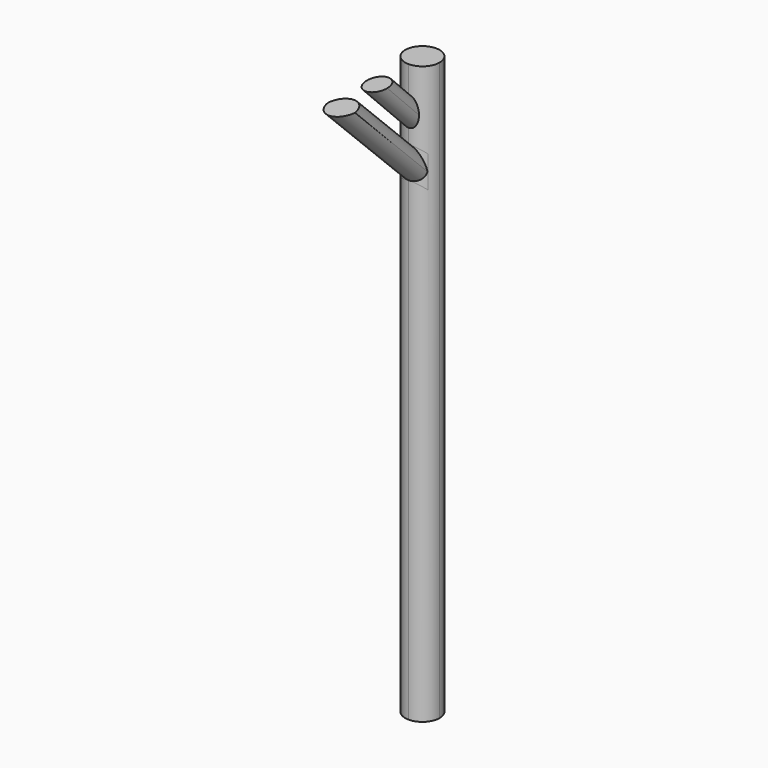
from build123d import *

# Parameters (mm, degrees)
F1_DEPTH     = 63.5
F2_DEPTH     = 38.1
F3_DEPTH     = 50.8
F4_T1_DEPTH  = 2451.0995000004
F4_T6_DEPTH  = 2451.0995000004
F4_T12_DEPTH = 2451.0995000004
F4_T18_DEPTH = 2451.0995000004
F4_T25_DEPTH = 2451.0995000004
F4_T31_DEPTH = 2451.0995000004
F4_T37_DEPTH = 2451.0995000004
F4_T43_DEPTH = 2451.0995000004
F4_T49_DEPTH = 2451.0995000004
F4_T56_DEPTH = 2451.0995000004
F4_T62_DEPTH = 2451.0995000004
F5_R         = 38.09999
F6_T3_DEPTH  = 804.0537236545
F6_S4_R      = 63.5000000002
F6_T5_DEPTH  = 430
F6_T8_DEPTH  = 804.0537236545
F6_S9_R      = 63.5000000002
F6_T10_DEPTH = 430
F6_T13_DEPTH = 641.6247372202
F6_S14_R     = 63.5000000002
F6_T15_DEPTH = 349
F6_T18_DEPTH = 641.6247372202
F6_S19_R     = 63.5000000002
F6_T20_DEPTH = 349
F6_T23_DEPTH = 641.6247372202
F6_S24_R     = 63.5000000002
F6_T25_DEPTH = 349
F6_T28_DEPTH = 641.6247372202
F6_S29_R     = 63.5000000002
F6_T30_DEPTH = 349
F6_T33_DEPTH = 804.0537236545
F6_S34_R     = 63.5000000002
F6_T35_DEPTH = 430
F6_T38_DEPTH = 804.0537236545
F6_S39_R     = 63.5000000002
F6_T40_DEPTH = 430


# Not quite as in the source:
# - a fillet or chamfer that OpenCascade refuses, or shapes differently, is made with other operations: its cross-section is extruded or revolved along the edge and cut away or added
# - a fillet or chamfer is up to 0.001 mm smaller than in the source, because OpenCascade refuses the exact size


with BuildPart() as f1:
    # F0 (on Right) → F1 (new body, symmetric)
    with BuildSketch(Plane.YZ):
        Polygon((-127, 1755.4620370299), (-127, 0), (0, 0), (0, 2133.6), (-127, 2133.6), (-127, 2034.3245418301), (-127, 1926.4060574944), (-127, 1872.7545669842), align=None)
    extrude(amount=F1_DEPTH, both=True)

    # F0 (on Right) → F3 (join, symmetric)
    with BuildSketch(Plane.YZ):
        Polygon((-495.5889745507, 2116.2556735062), (-127, 1755.4620370299), (-127, 1872.7545669842), (-379.5134473118, 2119.9275732464), align=None)
    extrude(amount=F3_DEPTH, both=True)

    # F4: fillet of radius 63.5 on 4 edges, made by hand

    # F4_s2 → F4_t1 (cut)
    with BuildSketch(Plane.XY.offset(-158.7497500002)):
        with BuildLine():
            ThreePointArc((-63.5001, -63.4999), (-44.9013806053, -18.5986193947), (-0.0001, 0.0001))
            Line((-0.0001, 0.0001), (-0.0001, 1.2701))
            Line((-0.0001, 1.2701), (-64.77, 1.27))
            Line((-64.77, 1.27), (-64.7701, -63.4999))
            Line((-64.7701, -63.4999), (-63.5001, -63.4999))
        make_face()
        with BuildLine():
            ThreePointArc((63.5001, -63.4999), (44.9013806053, -18.5986193947), (0.0001, 0.0001))
            Line((0.0001, 0.0001), (0.0001, 1.2701))
            Line((0.0001, 1.2701), (64.77, 1.27))
            Line((64.77, 1.27), (64.7701, -63.4999))
            Line((64.7701, -63.4999), (63.5001, -63.4999))
        make_face()
    extrude(amount=F4_T1_DEPTH, mode=Mode.SUBTRACT)


with BuildPart() as f2:
    # F0 (on Right) → F2 (new body, symmetric)
    with BuildSketch(Plane.YZ):
        Polygon((-326.3924083134, 2126.3731611819), (-127, 1926.4060574944), (-127, 2034.3245418301), (-220.5952878332, 2128.1895930882), align=None)
    extrude(amount=F2_DEPTH, both=True)

    # F5 (radius 38.1 in the source; OpenCascade refuses exactly that, so slightly less here)
    f5_edges = [f2.edges().sort_by_distance(p)[0] for p in [
        (-38.1, -226.696204, 2026.389609),
        (-38.1, -173.797644, 2081.257067),
        (38.1, -173.797644, 2081.257067),
        (38.1, -226.696204, 2026.389609),
    ]]
    fillet(f5_edges, radius=F5_R)


with BuildPart() as f4_tool4:
    # F4_s5 → F4_t6 (new body)
    with BuildSketch(Plane.XY.offset(2292.3497500002)):
        with BuildLine():
            ThreePointArc((-0.0001, -127.0001), (-44.9013806053, -108.4013806053), (-63.5001, -63.5001))
            Line((-63.5001, -63.5001), (-64.7701, -63.5001))
            Line((-64.7701, -63.5001), (-64.77, -128.27))
            Line((-64.77, -128.27), (-0.0001, -128.2701))
            Line((-0.0001, -128.2701), (-0.0001, -127.0001))
        make_face()
    extrude(amount=-F4_T6_DEPTH)

    split(bisect_by=Plane(origin=(0, 874.0205617241, 892.9047245081), x_dir=(1, 0, 0), z_dir=(0, 0.6995095685, 0.7146232319)), keep=Keep.TOP)

    split(bisect_by=Plane.YZ.offset(-50.8), keep=Keep.TOP)


with BuildPart() as f1_1:
    add(f1.part)

    # F4_t3: cut F4_tool4
    add(f4_tool4.part, mode=Mode.SUBTRACT)


with BuildPart() as f4_tool10:
    # F4_s11 → F4_t12 (new body)
    with BuildSketch(Plane.XY.offset(2292.3497500002)):
        with BuildLine():
            ThreePointArc((-0.0001, -127.0001), (-44.9013806053, -108.4013806053), (-63.5001, -63.5001))
            Line((-63.5001, -63.5001), (-64.7701, -63.5001))
            Line((-64.7701, -63.5001), (-64.77, -128.27))
            Line((-64.77, -128.27), (-0.0001, -128.2701))
            Line((-0.0001, -128.2701), (-0.0001, -127.0001))
        make_face()
    extrude(amount=-F4_T12_DEPTH)

    split(bisect_by=Plane(origin=(0, 874.0205617241, 892.9047245081), x_dir=(1, 0, 0), z_dir=(0, 0.6995095685, 0.7146232319)), keep=Keep.TOP)

    split(bisect_by=Plane.YZ.offset(-50.8), keep=Keep.BOTTOM)


with BuildPart() as f1_2:
    add(f1_1.part)

    # F4_t9: cut F4_tool10
    add(f4_tool10.part, mode=Mode.SUBTRACT)


with BuildPart() as f4_tool16:
    # F4_s17 → F4_t18 (new body)
    with BuildSketch(Plane.XY.offset(2292.3497500002)):
        with BuildLine():
            ThreePointArc((-0.0001, -127.0001), (-44.9013806053, -108.4013806053), (-63.5001, -63.5001))
            Line((-63.5001, -63.5001), (-64.7701, -63.5001))
            Line((-64.7701, -63.5001), (-64.77, -128.27))
            Line((-64.77, -128.27), (-0.0001, -128.2701))
            Line((-0.0001, -128.2701), (-0.0001, -127.0001))
        make_face()
    extrude(amount=-F4_T18_DEPTH)

    split(bisect_by=Plane(origin=(0, 874.0205617241, 892.9047245081), x_dir=(1, 0, 0), z_dir=(0, -0.6995095685, -0.7146232319)), keep=Keep.TOP)

    split(bisect_by=Plane.YZ.offset(-50.8), keep=Keep.BOTTOM)

    split(bisect_by=Plane(origin=(0, 815.3876928922, 833.0050289126), x_dir=(1, 0, 0), z_dir=(0, 0.6995095685, 0.7146232319)), keep=Keep.TOP)


with BuildPart() as f1_3:
    add(f1_2.part)

    # F4_t15: cut F4_tool16
    add(f4_tool16.part, mode=Mode.SUBTRACT)


with BuildPart() as f4_tool23:
    # F4_s24 → F4_t25 (new body)
    with BuildSketch(Plane.XY.offset(2292.3497500002)):
        with BuildLine():
            ThreePointArc((-0.0001, -127.0001), (-44.9013806053, -108.4013806053), (-63.5001, -63.5001))
            Line((-63.5001, -63.5001), (-64.7701, -63.5001))
            Line((-64.7701, -63.5001), (-64.77, -128.27))
            Line((-64.77, -128.27), (-0.0001, -128.2701))
            Line((-0.0001, -128.2701), (-0.0001, -127.0001))
        make_face()
    extrude(amount=-F4_T25_DEPTH)

    split(bisect_by=Plane.YZ.offset(-50.8), keep=Keep.TOP)

    split(bisect_by=Plane(origin=(0, 815.3876928922, 833.0050289126), x_dir=(1, 0, 0), z_dir=(0, -0.6995095685, -0.7146232319)), keep=Keep.TOP)


with BuildPart() as f1_4:
    add(f1_3.part)

    # F4_t22: cut F4_tool23
    add(f4_tool23.part, mode=Mode.SUBTRACT)


with BuildPart() as f4_tool29:
    # F4_s30 → F4_t31 (new body)
    with BuildSketch(Plane.XY.offset(2292.3497500002)):
        with BuildLine():
            ThreePointArc((-0.0001, -127.0001), (-44.9013806053, -108.4013806053), (-63.5001, -63.5001))
            Line((-63.5001, -63.5001), (-64.7701, -63.5001))
            Line((-64.7701, -63.5001), (-64.77, -128.27))
            Line((-64.77, -128.27), (-0.0001, -128.2701))
            Line((-0.0001, -128.2701), (-0.0001, -127.0001))
        make_face()
    extrude(amount=-F4_T31_DEPTH)

    split(bisect_by=Plane.YZ.offset(-50.8), keep=Keep.BOTTOM)

    split(bisect_by=Plane(origin=(0, 815.3876928922, 833.0050289126), x_dir=(1, 0, 0), z_dir=(0, -0.6995095685, -0.7146232319)), keep=Keep.TOP)


with BuildPart() as f1_5:
    add(f1_4.part)

    # F4_t28: cut F4_tool29
    add(f4_tool29.part, mode=Mode.SUBTRACT)


with BuildPart() as f4_tool35:
    # F4_s36 → F4_t37 (new body)
    with BuildSketch(Plane.XY.offset(-158.7497500002)):
        with BuildLine():
            ThreePointArc((0.0001, -127.0001), (44.9013806053, -108.4013806053), (63.5001, -63.5001))
            Line((63.5001, -63.5001), (64.7701, -63.5001))
            Line((64.7701, -63.5001), (64.77, -128.27))
            Line((64.77, -128.27), (0.0001, -128.2701))
            Line((0.0001, -128.2701), (0.0001, -127.0001))
        make_face()
    extrude(amount=F4_T37_DEPTH)

    split(bisect_by=Plane(origin=(0, 815.3876928922, 833.0050289126), x_dir=(1, 0, 0), z_dir=(0, -0.6995095685, -0.7146232319)), keep=Keep.TOP)

    split(bisect_by=Plane.YZ.offset(50.8), keep=Keep.BOTTOM)


with BuildPart() as f1_6:
    add(f1_5.part)

    # F4_t34: cut F4_tool35
    add(f4_tool35.part, mode=Mode.SUBTRACT)


with BuildPart() as f4_tool41:
    # F4_s42 → F4_t43 (new body)
    with BuildSketch(Plane.XY.offset(-158.7497500002)):
        with BuildLine():
            ThreePointArc((0.0001, -127.0001), (44.9013806053, -108.4013806053), (63.5001, -63.5001))
            Line((63.5001, -63.5001), (64.7701, -63.5001))
            Line((64.7701, -63.5001), (64.77, -128.27))
            Line((64.77, -128.27), (0.0001, -128.2701))
            Line((0.0001, -128.2701), (0.0001, -127.0001))
        make_face()
    extrude(amount=F4_T43_DEPTH)

    split(bisect_by=Plane(origin=(0, 815.3876928922, 833.0050289126), x_dir=(1, 0, 0), z_dir=(0, -0.6995095685, -0.7146232319)), keep=Keep.TOP)

    split(bisect_by=Plane.YZ.offset(50.8), keep=Keep.TOP)


with BuildPart() as f1_7:
    add(f1_6.part)

    # F4_t40: cut F4_tool41
    add(f4_tool41.part, mode=Mode.SUBTRACT)


with BuildPart() as f4_tool47:
    # F4_s48 → F4_t49 (new body)
    with BuildSketch(Plane.XY.offset(-158.7497500002)):
        with BuildLine():
            ThreePointArc((0.0001, -127.0001), (44.9013806053, -108.4013806053), (63.5001, -63.5001))
            Line((63.5001, -63.5001), (64.7701, -63.5001))
            Line((64.7701, -63.5001), (64.77, -128.27))
            Line((64.77, -128.27), (0.0001, -128.2701))
            Line((0.0001, -128.2701), (0.0001, -127.0001))
        make_face()
    extrude(amount=F4_T49_DEPTH)

    split(bisect_by=Plane(origin=(0, 874.0205617241, 892.9047245081), x_dir=(1, 0, 0), z_dir=(0, -0.6995095685, -0.7146232319)), keep=Keep.TOP)

    split(bisect_by=Plane(origin=(0, 815.3876928922, 833.0050289126), x_dir=(1, 0, 0), z_dir=(0, 0.6995095685, 0.7146232319)), keep=Keep.TOP)

    split(bisect_by=Plane.YZ.offset(50.8), keep=Keep.TOP)


with BuildPart() as f1_8:
    add(f1_7.part)

    # F4_t46: cut F4_tool47
    add(f4_tool47.part, mode=Mode.SUBTRACT)


with BuildPart() as f4_tool54:
    # F4_s55 → F4_t56 (new body)
    with BuildSketch(Plane.XY.offset(-158.7497500002)):
        with BuildLine():
            ThreePointArc((0.0001, -127.0001), (44.9013806053, -108.4013806053), (63.5001, -63.5001))
            Line((63.5001, -63.5001), (64.7701, -63.5001))
            Line((64.7701, -63.5001), (64.77, -128.27))
            Line((64.77, -128.27), (0.0001, -128.2701))
            Line((0.0001, -128.2701), (0.0001, -127.0001))
        make_face()
    extrude(amount=F4_T56_DEPTH)

    split(bisect_by=Plane(origin=(0, 874.0205617241, 892.9047245081), x_dir=(1, 0, 0), z_dir=(0, 0.6995095685, 0.7146232319)), keep=Keep.TOP)

    split(bisect_by=Plane.YZ.offset(50.8), keep=Keep.BOTTOM)


with BuildPart() as f1_9:
    add(f1_8.part)

    # F4_t53: cut F4_tool54
    add(f4_tool54.part, mode=Mode.SUBTRACT)


with BuildPart() as f4_tool60:
    # F4_s61 → F4_t62 (new body)
    with BuildSketch(Plane.XY.offset(-158.7497500002)):
        with BuildLine():
            ThreePointArc((0.0001, -127.0001), (44.9013806053, -108.4013806053), (63.5001, -63.5001))
            Line((63.5001, -63.5001), (64.7701, -63.5001))
            Line((64.7701, -63.5001), (64.77, -128.27))
            Line((64.77, -128.27), (0.0001, -128.2701))
            Line((0.0001, -128.2701), (0.0001, -127.0001))
        make_face()
    extrude(amount=F4_T62_DEPTH)

    split(bisect_by=Plane(origin=(0, 874.0205617241, 892.9047245081), x_dir=(1, 0, 0), z_dir=(0, 0.6995095685, 0.7146232319)), keep=Keep.TOP)

    split(bisect_by=Plane.YZ.offset(50.8), keep=Keep.TOP)


with BuildPart() as f1_10:
    add(f1_9.part)

    # F4_t59: cut F4_tool60
    add(f4_tool60.part, mode=Mode.SUBTRACT)

    # F6: fillet of radius 50.546 on 4 edges, made by hand


with BuildPart() as f6_tool1:
    # F6_s2 → F6_t3 (new body)
    with BuildSketch(Plane(origin=(0, -826.6845615268, 809.2008979259), x_dir=(1, 0, 0), z_dir=(0, -0.7146232319, 0.6995095685))):
        with BuildLine():
            ThreePointArc((-50.8, 1216.2022391691), (-35.9954193619, 1180.4608198072), (-0.254, 1165.6562391691))
            Line((-0.254, 1165.6562391691), (-50.8, 1165.6562391691))
            Line((-50.8, 1165.6562391691), (-50.8, 1216.2022391691))
        make_face()
    extrude(amount=F6_T3_DEPTH)

    # F6_s4 → F6_t5 (cut, symmetric)
    with BuildSketch(Plane.XY.offset(1941.5)):
        with Locations((-9.99998e-05, -63.5000999998)):
            Circle(F6_S4_R)
    extrude(amount=F6_T5_DEPTH, both=True, mode=Mode.SUBTRACT)


with BuildPart() as f6_tool6:
    # F6_s7 → F6_t8 (new body)
    with BuildSketch(Plane(origin=(0, -826.6845615268, 809.2008979259), x_dir=(1, 0, 0), z_dir=(0, -0.7146232319, 0.6995095685))):
        with BuildLine():
            ThreePointArc((-50.8, 1216.2022391691), (-35.9954193619, 1180.4608198072), (-0.254, 1165.6562391691))
            Line((-0.254, 1165.6562391691), (-50.8, 1165.6562391691))
            Line((-50.8, 1165.6562391691), (-50.8, 1216.2022391691))
        make_face()
    extrude(amount=F6_T8_DEPTH)

    # F6_s9 → F6_t10 (cut, symmetric)
    with BuildSketch(Plane.XY.offset(1941.5)):
        with Locations((-9.99998e-05, -63.4999000002)):
            Circle(F6_S9_R)
    extrude(amount=F6_T10_DEPTH, both=True, mode=Mode.SUBTRACT)


with BuildPart() as f6_tool11:
    # F6_s12 → F6_t13 (new body)
    with BuildSketch(Plane(origin=(0, -1343.8373737342, 1315.416375363), x_dir=(1, 0, 0), z_dir=(0, 0.7146232319, -0.6995095685))):
        with BuildLine():
            ThreePointArc((-50.8, -1198.9302060021), (-35.9954193619, -1234.671625364), (-0.254, -1249.4762060021))
            Line((-0.254, -1249.4762060021), (-50.8, -1249.4762060021))
            Line((-50.8, -1249.4762060021), (-50.8, -1198.9302060021))
        make_face()
    extrude(amount=F6_T13_DEPTH)

    # F6_s14 → F6_t15 (cut, symmetric)
    with BuildSketch(Plane.XY.offset(1965.8)):
        with Locations((-9.99998e-05, -63.4999000002)):
            Circle(F6_S14_R)
    extrude(amount=F6_T15_DEPTH, both=True, mode=Mode.SUBTRACT)


with BuildPart() as f6_tool16:
    # F6_s17 → F6_t18 (new body)
    with BuildSketch(Plane(origin=(0, -1343.8373737342, 1315.416375363), x_dir=(1, 0, 0), z_dir=(0, 0.7146232319, -0.6995095685))):
        with BuildLine():
            ThreePointArc((-50.8, -1198.9302060021), (-35.9954193619, -1234.671625364), (-0.254, -1249.4762060021))
            Line((-0.254, -1249.4762060021), (-50.8, -1249.4762060021))
            Line((-50.8, -1249.4762060021), (-50.8, -1198.9302060021))
        make_face()
    extrude(amount=F6_T18_DEPTH)

    # F6_s19 → F6_t20 (cut, symmetric)
    with BuildSketch(Plane.XY.offset(1965.8)):
        with Locations((-9.99998e-05, -63.5000999998)):
            Circle(F6_S19_R)
    extrude(amount=F6_T20_DEPTH, both=True, mode=Mode.SUBTRACT)


with BuildPart() as f6_tool21:
    # F6_s22 → F6_t23 (new body)
    with BuildSketch(Plane(origin=(0, -1343.8373737342, 1315.416375363), x_dir=(1, 0, 0), z_dir=(0, 0.7146232319, -0.6995095685))):
        with BuildLine():
            ThreePointArc((50.8, -1198.9302060021), (35.9954193619, -1234.671625364), (0.254, -1249.4762060021))
            Line((0.254, -1249.4762060021), (50.8, -1249.4762060021))
            Line((50.8, -1249.4762060021), (50.8, -1198.9302060021))
        make_face()
    extrude(amount=F6_T23_DEPTH)

    # F6_s24 → F6_t25 (cut, symmetric)
    with BuildSketch(Plane.XY.offset(1965.8)):
        with Locations((9.99998e-05, -63.4999000002)):
            Circle(F6_S24_R)
    extrude(amount=F6_T25_DEPTH, both=True, mode=Mode.SUBTRACT)


with BuildPart() as f6_tool26:
    # F6_s27 → F6_t28 (new body)
    with BuildSketch(Plane(origin=(0, -1343.8373737342, 1315.416375363), x_dir=(1, 0, 0), z_dir=(0, 0.7146232319, -0.6995095685))):
        with BuildLine():
            ThreePointArc((50.8, -1198.9302060021), (35.9954193619, -1234.671625364), (0.254, -1249.4762060021))
            Line((0.254, -1249.4762060021), (50.8, -1249.4762060021))
            Line((50.8, -1249.4762060021), (50.8, -1198.9302060021))
        make_face()
    extrude(amount=F6_T28_DEPTH)

    # F6_s29 → F6_t30 (cut, symmetric)
    with BuildSketch(Plane.XY.offset(1965.8)):
        with Locations((9.99998e-05, -63.5000999998)):
            Circle(F6_S29_R)
    extrude(amount=F6_T30_DEPTH, both=True, mode=Mode.SUBTRACT)


with BuildPart() as f6_tool31:
    # F6_s32 → F6_t33 (new body)
    with BuildSketch(Plane(origin=(0, -826.6845615268, 809.2008979259), x_dir=(1, 0, 0), z_dir=(0, -0.7146232319, 0.6995095685))):
        with BuildLine():
            ThreePointArc((50.8, 1216.2022391691), (35.9954193619, 1180.4608198072), (0.254, 1165.6562391691))
            Line((0.254, 1165.6562391691), (50.8, 1165.6562391691))
            Line((50.8, 1165.6562391691), (50.8, 1216.2022391691))
        make_face()
    extrude(amount=F6_T33_DEPTH)

    # F6_s34 → F6_t35 (cut, symmetric)
    with BuildSketch(Plane.XY.offset(1941.5)):
        with Locations((9.99998e-05, -63.5000999998)):
            Circle(F6_S34_R)
    extrude(amount=F6_T35_DEPTH, both=True, mode=Mode.SUBTRACT)


with BuildPart() as f6_tool36:
    # F6_s37 → F6_t38 (new body)
    with BuildSketch(Plane(origin=(0, -826.6845615268, 809.2008979259), x_dir=(1, 0, 0), z_dir=(0, -0.7146232319, 0.6995095685))):
        with BuildLine():
            ThreePointArc((50.8, 1216.2022391691), (35.9954193619, 1180.4608198072), (0.254, 1165.6562391691))
            Line((0.254, 1165.6562391691), (50.8, 1165.6562391691))
            Line((50.8, 1165.6562391691), (50.8, 1216.2022391691))
        make_face()
    extrude(amount=F6_T38_DEPTH)

    # F6_s39 → F6_t40 (cut, symmetric)
    with BuildSketch(Plane.XY.offset(1941.5)):
        with Locations((9.99998e-05, -63.4999000002)):
            Circle(F6_S39_R)
    extrude(amount=F6_T40_DEPTH, both=True, mode=Mode.SUBTRACT)


with BuildPart() as f1_11:
    add(f1_10.part)

    # F6_t41: cut F6_tool1, F6_tool6, F6_tool11, F6_tool16, F6_tool21, F6_tool26, F6_tool31, F6_tool36
    add([f6_tool1.part, f6_tool6.part, f6_tool11.part, f6_tool16.part, f6_tool21.part, f6_tool26.part, f6_tool31.part, f6_tool36.part], mode=Mode.SUBTRACT)


solid = Compound([f2.part, f1_11.part])
